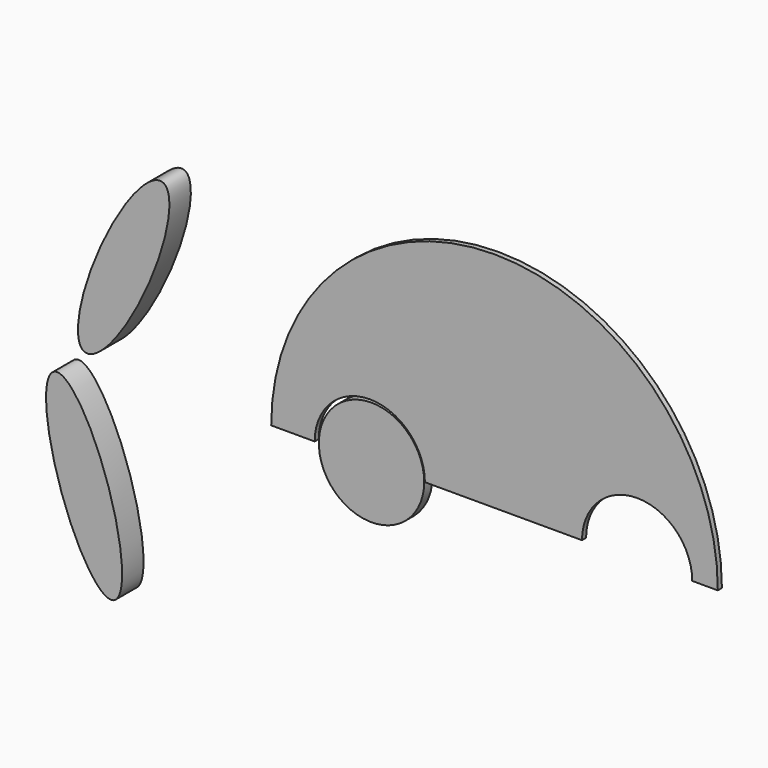
from build123d import *

# Parameters (mm, degrees)
F3_DEPTH  = 1.016
F8_DEPTH  = 5.334
F9_R      = 10.4858478574
F10_DEPTH = 2.032


# Not quite as in the source:
# - the program builds the solid bodies; features that only make, move or delete a surface that nothing else refers to are left out


with BuildPart() as f3:
    # F0 (on Front) → F3 (new body)
    with BuildSketch(Plane.XZ):
        with BuildLine():
            Line((39.4395558923, 0), (44.5358680129, 0))
            ThreePointArc((44.5358680129, 0), (0.0858680129, 44.45), (-44.3641319871, 0))
            Line((-44.3641319871, 0), (-35.7163650749, 0))
            ThreePointArc((-35.7163650749, 0), (-24.7461050749, 10.97026), (-13.7758450749, 0))
            Line((-13.7758450749, 0), (17.4985149116, 0))
            ThreePointArc((17.4985149116, 0), (28.4690354019, 10.9705204904), (39.4395558923, 0))
        make_face()
    extrude(amount=-F3_DEPTH)


with BuildPart() as f8:
    # F7 (on Front) → F8 (new body)
    with BuildSketch(Plane.XZ):
        with BuildLine():
            add(Edge.make_bspline(
                [(-71.5328833988, -37.3046489378), (-63.153925009, -34.6190845086), (-76.0650305258, -8.7504011379), (-88.9761360426, 17.1182822328), (-84.4439889156, -11.4359655671), (-79.9118417885, -39.990213367), (-71.5328833988, -37.3046489378)],
                knots=[0, 0, 0, 2.0943951024, 2.0943951024, 4.1887902048, 4.1887902048, 6.2831853072, 6.2831853072, 6.2831853072], degree=2, weights=[1, 0.5, 1, 0.5, 1, 0.5, 1]))
        make_face()
    extrude(amount=F8_DEPTH)


with BuildPart() as f8b:
    # F7 (on Front) → F8, piece 2 (new body)
    with BuildSketch(Plane.XZ):
        with BuildLine():
            add(Edge.make_bspline(
                [(-61.6284896097, 39.1108230438), (-69.648656578, 42.7296794653), (-77.3911540702, 14.8739949901), (-85.1336515623, -12.9816894852), (-69.3709871018, 11.2551385686), (-53.6083226413, 35.4919666223), (-61.6284896097, 39.1108230438)],
                knots=[0, 0, 0, 2.0943951024, 2.0943951024, 4.1887902048, 4.1887902048, 6.2831853072, 6.2831853072, 6.2831853072], degree=2, weights=[1, 0.5, 1, 0.5, 1, 0.5, 1]))
        make_face()
    extrude(amount=F8_DEPTH)


with BuildPart() as f10:
    # F9 (on Front) → F10 (new body)
    with BuildSketch(Plane.XZ):
        with Locations((-24.3968013674, 0)):
            Circle(F9_R)
    extrude(amount=-F10_DEPTH)


solid = Compound([f3.part, f8.part, f8b.part, f10.part])
